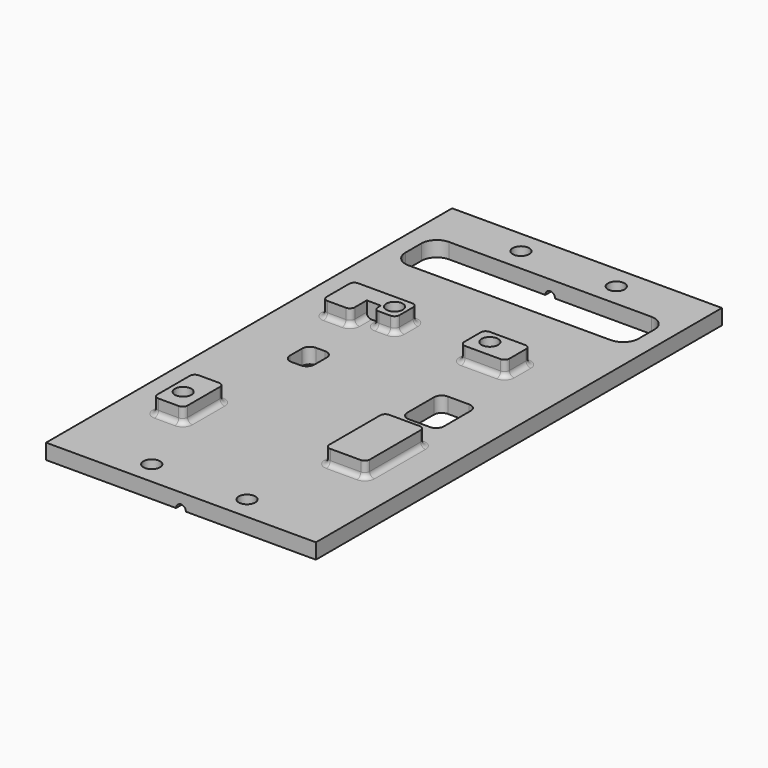
from build123d import *

# Parameters (mm, degrees)
F0_W     = 55.88
F0_H     = 105.1052
F0_R     = 1.7145
F0_W_2   = 48.26
F0_H_2   = 10.4902
F1_DEPTH = 3.175
F2_R     = 1.016
F3_DEPTH = 105.1062
F4_R     = 1.7145
F4_W     = 9.3726
F4_H     = 6.35
F4_W_2   = 6.223
F4_H_2   = 10.414
F4_W_3   = 8.3566
F4_H_3   = 15.24
F5_DEPTH = 3.175
F6_W     = 7.62
F6_H     = 10.16
F6_W_2   = 5.08
F6_H_2   = 6.35
F7_DEPTH = 25.4
F8_R     = 1.6002
F9_R     = 3.175
F10_F1_R = 1.016
F10_F2_R = 1.016


# Not quite as in the source:
# - a feature names something its author has since deleted; it is built from what else it names


with BuildPart() as f1:
    # F0 (on Top) → F1 (new body)
    with BuildSketch(Plane.XY):
        Rectangle(F0_W, F0_H)
        with Locations((-17.9451, -29.5656)):
            Circle(F0_R, mode=Mode.SUBTRACT)
        with Locations((-9.8679, -47.7901)):
            Circle(F0_R, mode=Mode.SUBTRACT)
        with Locations((9.8679, -47.7901)):
            Circle(F0_R, mode=Mode.SUBTRACT)
        with Locations((-9.8679, 15.0622)):
            Circle(F0_R, mode=Mode.SUBTRACT)
        with Locations((0, 37.7825)):
            Rectangle(F0_W_2, F0_H_2, mode=Mode.SUBTRACT)
        with Locations((-9.8679, 47.7901)):
            Circle(F0_R, mode=Mode.SUBTRACT)
        with Locations((9.8679, 15.0622)):
            Circle(F0_R, mode=Mode.SUBTRACT)
        with Locations((9.8679, 47.7901)):
            Circle(F0_R, mode=Mode.SUBTRACT)
    extrude(amount=F1_DEPTH)

    # F2 (on face) → F3 (cut, through all)
    with BuildSketch(Plane.XZ.offset(52.5526)):
        Circle(F2_R)
    extrude(amount=-F3_DEPTH, mode=Mode.SUBTRACT)

    # F4 (on face) → F5 (join)
    with BuildSketch(Plane.XY.offset(3.175)):
        Polygon((-7.3914, 17.7927), (-20.5994, 17.7927), (-20.5994, 14.8093839596), (-20.5994, 9.8679), (-14.7574, 9.8679), (-14.7574, 13.9827), (-11.8364, 13.9827), (-11.8364, 12.2047), (-7.3914, 12.2047), (-7.3914, 13.9827), align=None)
        with Locations((-9.8679, 15.0622)):
            Circle(F4_R, mode=Mode.SUBTRACT)
        with Locations((11.3157, 14.6177)):
            Rectangle(F4_W, F4_H)
        with Locations((9.8679, 15.0622)):
            Circle(F4_R, mode=Mode.SUBTRACT)
        with Locations((-17.4879, -28.6893)):
            Rectangle(F4_W_2, F4_H_2)
        with Locations((-17.9451, -29.5656)):
            Circle(F4_R, mode=Mode.SUBTRACT)
        with Locations((16.2687, -22.6695)):
            Rectangle(F4_W_3, F4_H_3)
    extrude(amount=F5_DEPTH)

    # F6 (on face) → F7 (cut)
    with BuildSketch(Plane(origin=(0, 0, 0), x_dir=(1, 0, 0), z_dir=(0, 0, -1))):
        with Locations((14.9225, 4.4323)):
            Rectangle(F6_W, F6_H)
        with Locations((-13.6525, 2.5273)):
            Rectangle(F6_W_2, F6_H_2)
    extrude(amount=-F7_DEPTH, mode=Mode.SUBTRACT)

    # F8
    f8_edges = [f1.edges().sort_by_distance(p)[0] for p in [
        (-16.1925, 0.6477, 1.5875),
        (11.1125, 0.6477, 1.5875),
        (18.7325, 0.6477, 1.5875),
        (18.7325, -9.5123, 1.5875),
        (11.1125, -9.5123, 1.5875),
        (-16.1925, -5.7023, 1.5875),
        (-11.1125, -5.7023, 1.5875),
        (-11.1125, 0.6477, 1.5875),
    ]]
    fillet(f8_edges, radius=F8_R)

    # F9
    f9_edges = [f1.edges().sort_by_distance(p)[0] for p in [
        (-24.13, 32.5374, 1.5875),
        (24.13, 32.5374, 1.5875),
        (24.13, 43.0276, 1.5875),
        (-24.13, 43.0276, 1.5875),
    ]]
    fillet(f9_edges, radius=F9_R)

    # F10: fillet of radius 1.016 on 34 edges, made by hand

    # F10_f1
    f10_f1_edges = [f1.edges().sort_by_distance(p)[0] for p in [
        (-7.3914, 17.7927, 4.7625),
        (6.6294, 17.7927, 4.7625),
        (16.002, 17.7927, 4.7625),
        (20.447, -15.0495, 4.7625),
        (12.0904, -15.0495, 4.7625),
        (20.447, -30.2895, 4.7625),
        (12.0904, -30.2895, 4.7625),
        (-14.3764, -33.8963, 4.7625),
        (-20.5994, -33.8963, 4.7625),
        (-14.3764, -23.4823, 4.7625),
        (-20.5994, -23.4823, 4.7625),
        (6.6294, 11.4427, 4.7625),
        (16.002, 11.4427, 4.7625),
        (-20.5994, 17.7927, 4.7625),
        (-20.5994, 9.8679, 4.7625),
        (-14.7574, 9.8679, 4.7625),
        (-7.3914, 12.2047, 4.7625),
        (-11.8364, 12.2047, 4.7625),
    ]]
    fillet(f10_f1_edges, radius=F10_F1_R)

    # F10_f2
    f10_f2_edges = [f1.edges().sort_by_distance(p)[0] for p in [
        (-14.3764, -28.6893, 3.175),
        (20.447, -22.6695, 3.175),
        (16.002, 14.6177, 3.175),
        (-7.3914, 14.9987, 3.175),
        (-20.5994, -28.6893, 3.175),
        (-17.4879, -23.4823, 3.175),
        (-17.4879, -33.8963, 3.175),
        (16.2687, -30.2895, 3.175),
        (16.2687, -15.0495, 3.175),
        (12.0904, -22.6695, 3.175),
        (-13.9954, 17.7927, 3.175),
        (-20.5994, 13.8303, 3.175),
        (-17.6784, 9.8679, 3.175),
        (11.3157, 11.4427, 3.175),
        (11.3157, 17.7927, 3.175),
        (6.6294, 14.6177, 3.175),
        (6.9269795103, 17.4951204897, 3.175),
        (6.9269795103, 11.7402795103, 3.175),
        (15.7044204897, 17.4951204897, 3.175),
        (15.7044204897, 11.7402795103, 3.175),
        (-20.3018204897, 10.1654795103, 3.175),
        (-15.0549795103, 10.1654795103, 3.175),
        (-20.3018204897, 17.4951204897, 3.175),
        (-7.6889795103, 17.4951204897, 3.175),
        (12.3879795103, -15.3470795103, 3.175),
        (12.3879795103, -29.9919204897, 3.175),
        (20.1494204897, -15.3470795103, 3.175),
        (20.1494204897, -29.9919204897, 3.175),
        (-20.3018204897, -33.5987204897, 3.175),
        (-14.6739795103, -33.5987204897, 3.175),
        (-14.6739795103, -23.7798795103, 3.175),
        (-20.3018204897, -23.7798795103, 3.175),
        (-7.6889795103, 12.5022795103, 3.175),
    ]]
    fillet(f10_f2_edges, radius=F10_F2_R)


solid = f1.part
